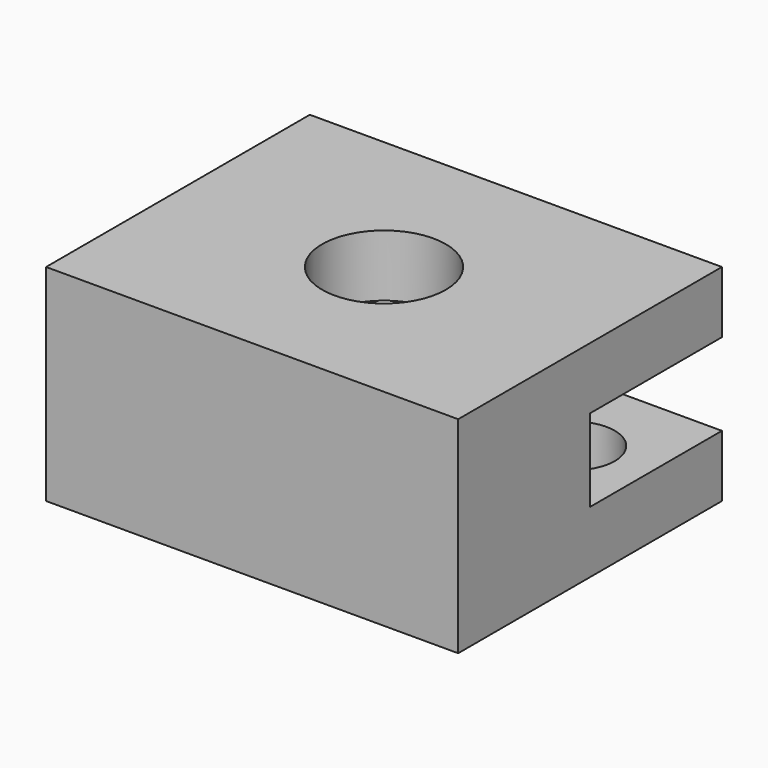
from build123d import *

# Parameters (mm, degrees)
F0_W     = 100
F0_H     = 80
F0_R     = 15
F1_DEPTH = 50
F2_W     = 100
F2_H     = 20
F3_DEPTH = 50
F4_R     = 10
F5_DEPTH = 15


# Not quite as in the source:
# - a pattern or mirror of a feature is missing from the dataset's text; its kind, count and spacing are read off the source's solid


with BuildPart() as f1:
    # F0 (on Top) → F1 (new body)
    with BuildSketch(Plane.XY):
        Rectangle(F0_W, F0_H)
        Circle(F0_R, mode=Mode.SUBTRACT)
    extrude(amount=F1_DEPTH)

    # F2 (on Front) → F3 (cut)
    with BuildSketch(Plane.XZ):
        with Locations((0, 25)):
            Rectangle(F2_W, F2_H)
    extrude(amount=-F3_DEPTH, mode=Mode.SUBTRACT)

    # F4 (on face) → F5 (cut, through all)
    with BuildSketch(Plane.XY.offset(15)):
        with Locations((31.9020673633, 17.6108591259)):
            Circle(F4_R)
    f5 = extrude(amount=-F5_DEPTH, mode=Mode.SUBTRACT)

    # F5_copies: F5 across plane
    add(f5.mirror(Plane(origin=(0, 0, 0), x_dir=(0, 0, -1), z_dir=(-1, 0, 0))), mode=Mode.SUBTRACT)


solid = f1.part
